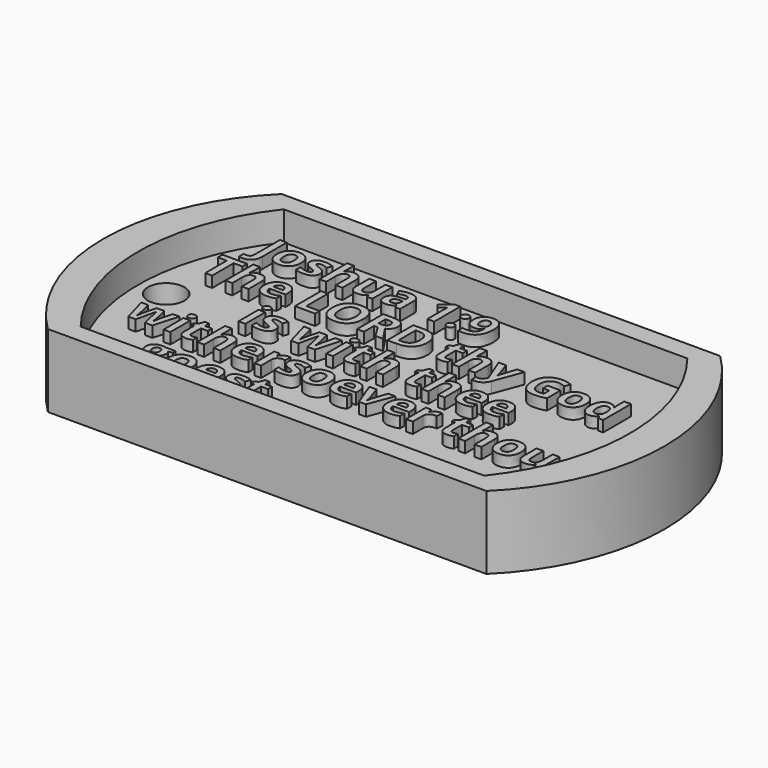
from build123d import *

# Parameters (mm, degrees)
F1_DEPTH     = 6.35
F2_DEPTH     = 3.81
F3_TEXT_SIZE = 3.96875
F4_DEPTH     = 0.9525
F5_R         = 1.5875
F6_DEPTH     = 25.4


# Not quite as in the source:
# - Text() gives the source's letters only with a copy of the font that has no kerning and outlines rounded to 1/6400 em; it was checked with that copy


with BuildPart() as f1:
    # F0 (on Top) → F1 (new body)
    with BuildSketch(Plane.XY):
        with BuildLine():
            Line((-19.05, -12.7), (19.05, -12.7))
            ThreePointArc((19.05, -12.7), (24.3865921067, 0), (19.05, 12.7))
            Line((19.05, 12.7), (-19.05, 12.7))
            ThreePointArc((-19.05, 12.7), (-24.3865921067, 0), (-19.05, -12.7))
        make_face()
        with BuildLine():
            ThreePointArc((17.5362508744, 11.0319061205), (21.3725982916, 0), (17.5362508744, -11.0319061205))
            Line((17.5362508744, -11.0319061205), (-17.5362508744, -11.0319061205))
            ThreePointArc((-17.5362508744, -11.0319061205), (-21.3725982916, 0), (-17.5362508744, 11.0319061205))
            Line((-17.5362508744, 11.0319061205), (17.5362508744, 11.0319061205))
        make_face(mode=Mode.SUBTRACT)
    extrude(amount=F1_DEPTH)

    # F0 (on Top) → F2 (join)
    with BuildSketch(Plane.XY):
        with BuildLine():
            Line((-17.5362508744, -11.0319061205), (17.5362508744, -11.0319061205))
            ThreePointArc((17.5362508744, -11.0319061205), (21.3725982916, 0), (17.5362508744, 11.0319061205))
            Line((17.5362508744, 11.0319061205), (-17.5362508744, 11.0319061205))
            ThreePointArc((-17.5362508744, 11.0319061205), (-21.3725982916, 0), (-17.5362508744, -11.0319061205))
        make_face()
    extrude(amount=F2_DEPTH)

    # F3 (on face) → F4 (join)
    with BuildSketch(Plane.XY.offset(3.81)):
        with Locations((-17.1900386613, 6.9044061205)):
            Text('Joshua 1:9', F3_TEXT_SIZE, font='Open Sans', font_style=FontStyle.BOLD, text_align=(TextAlign.LEFT, TextAlign.BOTTOM))
        with Locations((-11.8699645545, -1.3505938795)):
            Text('is with thee', F3_TEXT_SIZE, font='Open Sans', font_style=FontStyle.BOLD, text_align=(TextAlign.LEFT, TextAlign.BOTTOM))
        with Locations((-18.6009407043, 2.7769061205)):
            Text('The LORD thy God', F3_TEXT_SIZE, font='Open Sans', font_style=FontStyle.BOLD, text_align=(TextAlign.LEFT, TextAlign.BOTTOM))
        with Locations((-18.4818208218, -5.4780938795)):
            Text('withersoever thou', F3_TEXT_SIZE, font='Open Sans', font_style=FontStyle.BOLD, text_align=(TextAlign.LEFT, TextAlign.BOTTOM))
        with Locations((-14.3586373888, -9.6055938795)):
            Text('goest.', F3_TEXT_SIZE, font='Open Sans', font_style=FontStyle.BOLD, text_align=(TextAlign.LEFT, TextAlign.BOTTOM))
    extrude(amount=F4_DEPTH)

    # F5 (on face) → F6 (cut)
    with BuildSketch(Plane.XY.offset(3.81)):
        with Locations((-19.05, 0.1510304635)):
            Circle(F5_R)
    extrude(amount=-F6_DEPTH, mode=Mode.SUBTRACT)


solid = f1.part
